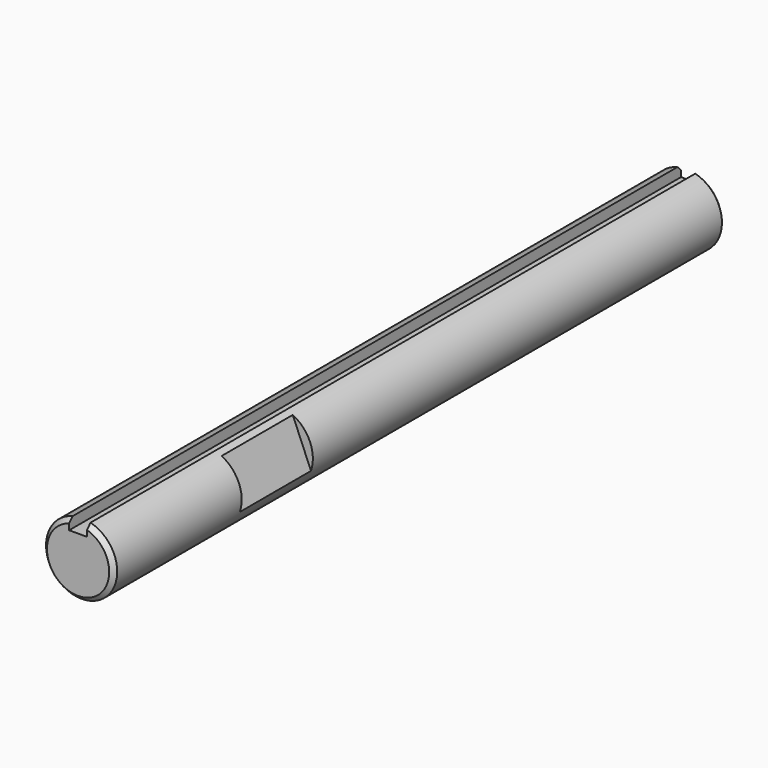
from build123d import *

# Parameters (mm, degrees)
F0_R     = 4
F1_DEPTH = 86
F2_W     = 2
F2_H     = 2.6729833462
F3_DEPTH = 86.001
F4_SIZE  = 0.5
F7_W     = 10
F7_H     = 16.0862193677
F8_DEPTH = 2.1892940191


with BuildPart() as f1:
    # F0 (on Front) → F1 (new body)
    with BuildSketch(Plane.XZ):
        Circle(F0_R)
    extrude(amount=F1_DEPTH)

    # F2 (on face) → F3 (cut, through all)
    with BuildSketch(Plane.XZ.offset(86)):
        with Locations((0, 4.0094750193)):
            Rectangle(F2_W, F2_H)
    extrude(amount=-F3_DEPTH, mode=Mode.SUBTRACT)

    # F4
    f4_edges = [f1.edges().sort_by_distance(p)[0] for p in [
        (0, -86, -4),
        (0, 0, -4),
    ]]
    chamfer(f4_edges, length=F4_SIZE)

    # F7 (on face) → F8 (cut, through all)
    with BuildSketch(Plane(origin=(2.7655894548, 0, 1.1625467594), x_dir=(0, -1, 0), z_dir=(-0.9218631516, 0, -0.3875155865))):
        with Locations((63, 0.6007021293)):
            Rectangle(F7_W, F7_H)
    extrude(amount=-F8_DEPTH, mode=Mode.SUBTRACT)


solid = f1.part
